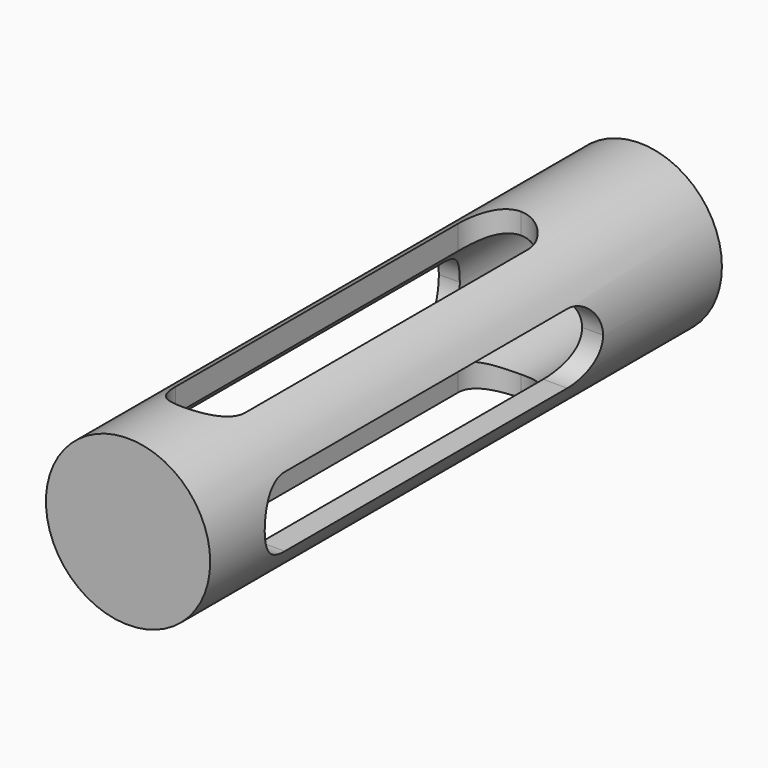
from build123d import *

# Parameters (mm, degrees)
F0_R     = 4.7
F1_DEPTH = 36.6
F2_R     = 3.5
F3_DEPTH = 34.5
F4_W     = 4
F4_H     = 24.2
F5_DEPTH = 12.5
F6_W     = 24.2
F6_H     = 4
F7_DEPTH = 12.5
F8_R     = 1.9999


# Not quite as in the source:
# - a fillet or chamfer is up to 0.001 mm smaller than in the source, because OpenCascade refuses the exact size


with BuildPart() as f1:
    # F0 (on Front) → F1 (new body)
    with BuildSketch(Plane.XZ):
        Circle(F0_R)
    extrude(amount=F1_DEPTH)

    # F2 (on face) → F3 (cut)
    with BuildSketch(Plane(origin=(0, 0, 0), x_dir=(-1, 0, 0), z_dir=(0, 1, 0))):
        Circle(F2_R)
    extrude(amount=-F3_DEPTH, mode=Mode.SUBTRACT)

    # F4 (on Top) → F5 (cut, symmetric)
    with BuildSketch(Plane.XY):
        with Locations((0, -20.6)):
            Rectangle(F4_W, F4_H)
    extrude(amount=F5_DEPTH, both=True, mode=Mode.SUBTRACT)

    # F6 (on Right) → F7 (cut, symmetric)
    with BuildSketch(Plane.YZ):
        with Locations((-20.6, 0)):
            Rectangle(F6_W, F6_H)
    extrude(amount=F7_DEPTH, both=True, mode=Mode.SUBTRACT)

    # F8 (radius 2 in the source; OpenCascade refuses exactly that, so slightly less here)
    f8_edges = [f1.edges().sort_by_distance(p)[0] for p in [
        (2, -8.5, 3.562758),
        (2, -8.5, -3.562758),
        (-2, -8.5, 3.562758),
        (-2, -8.5, -3.562758),
        (3.562758, -8.5, -2),
        (-3.562758, -8.5, -2),
        (3.562758, -8.5, 2),
        (-3.562758, -8.5, 2),
        (3.562758, -32.7, 2),
        (-3.562758, -32.7, 2),
        (3.562758, -32.7, -2),
        (-3.562758, -32.7, -2),
        (-2, -32.7, 3.562758),
        (-2, -32.7, -3.562758),
        (2, -32.7, 3.562758),
        (2, -32.7, -3.562758),
    ]]
    fillet(f8_edges, radius=F8_R)


solid = f1.part
